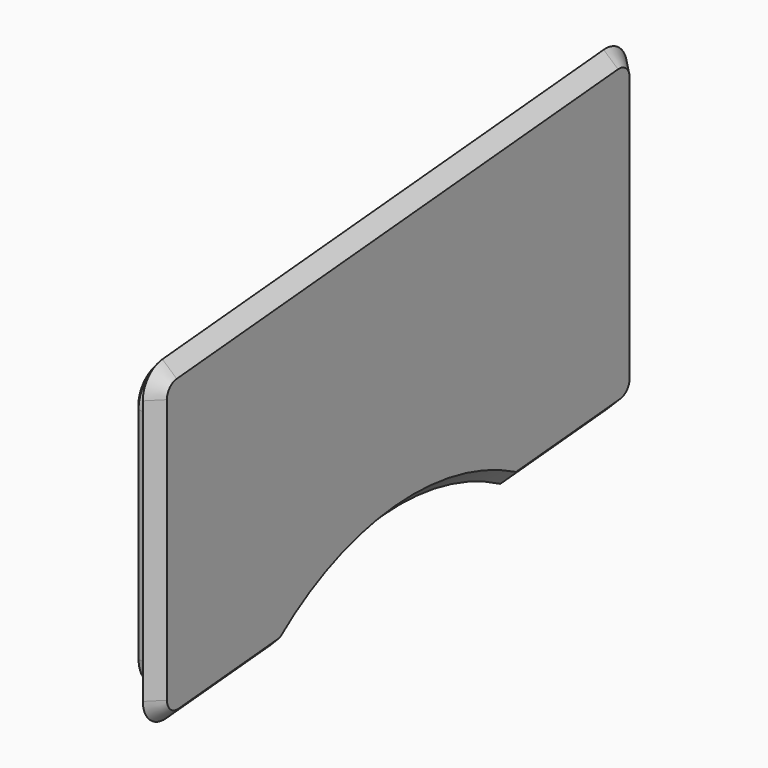
from build123d import *

# Parameters (mm, degrees)
F1_DEPTH     = 3
F2_DEPTH     = 8
F3_R         = 8
F4_T4_DEPTH  = 113.9006842239
F4_T9_ANGLE  = 95
F4_T14_ANGLE = 85
F4_T19_DEPTH = 49.1871720396
F4_T24_ANGLE = 95
F4_T29_DEPTH = 20.662188907
F4_T34_ANGLE = 31.4669762933
F4_T39_ANGLE = 62.9339525865
F4_T44_ANGLE = 31.4669762933
F4_T49_DEPTH = 22.2455379196
F4_T54_ANGLE = 85
F4_T59_DEPTH = 49.1871720396
F5_SIZE      = 1
F6_T1_DEPTH  = 123.9388825993
F6_T3_DEPTH  = 59.2253704151
F6_T5_DEPTH  = 42.8508484491
F6_T7_DEPTH  = 59.2253704151
F6_T9_DEPTH  = 43.5593108265
F6_T12_ANGLE = 96.9904356043
F6_T14_ANGLE = 95
F6_T16_ANGLE = 85
F6_T18_ANGLE = 95
F6_T20_ANGLE = 85


# Not quite as in the source:
# - a fillet or chamfer that OpenCascade refuses, or shapes differently, is made with other operations: its cross-section is extruded or revolved along the edge and cut away or added


with BuildPart() as f1:
    # F0 (on Right) → F1 (new body)
    with BuildSketch(Plane.YZ):
        with BuildLine():
            Line((-76.6886542646, 55.3186824411), (-76.6886542646, -19.9678053747))
            Line((-76.6886542646, -19.9678053747), (-38.1131050777, -16.5928821315))
            ThreePointArc((-38.1131050777, -16.5928821315), (-7.4822201157, -3.8748285682), (24.8917797013, -11.0806689666))
            Line((24.8917797013, -11.0806689666), (62.7786034683, -7.76600139))
            Line((62.7786034683, -7.76600139), (62.7786034683, 67.5204864257))
            Line((62.7786034683, 67.5204864257), (-76.6886542646, 55.3186824411))
        make_face()
        with BuildLine():
            Line((-40.0864817191, -11.7464310288), (-71.6886542646, -14.5112628693))
            Line((-71.6886542646, -14.5112628693), (-71.6886542646, 50.737026571))
            Line((-71.6886542646, 50.737026571), (57.7786034683, 62.0639439204))
            Line((57.7786034683, 62.0639439204), (57.7786034683, -3.1843455199))
            Line((57.7786034683, -3.1843455199), (25.9935989152, -5.9651730884))
            ThreePointArc((25.9935989152, -5.9651730884), (-7.9179988294, 1.1061449223), (-40.0864817191, -11.7464310288))
        make_face(mode=Mode.SUBTRACT)
        with BuildLine():
            Line((-71.6886542646, 50.737026571), (-71.6886542646, -14.5112628693))
            Line((-71.6886542646, -14.5112628693), (-40.0864817191, -11.7464310288))
            ThreePointArc((-40.0864817191, -11.7464310288), (-7.9179988294, 1.1061449223), (25.9935989152, -5.9651730884))
            Line((25.9935989152, -5.9651730884), (57.7786034683, -3.1843455199))
            Line((57.7786034683, -3.1843455199), (57.7786034683, 62.0639439204))
            Line((57.7786034683, 62.0639439204), (-71.6886542646, 50.737026571))
        make_face()
    extrude(amount=-F1_DEPTH)

    # F0 (on Right) → F2 (join)
    with BuildSketch(Plane.YZ):
        with BuildLine():
            Line((-71.6886542646, 50.737026571), (-71.6886542646, -14.5112628693))
            Line((-71.6886542646, -14.5112628693), (-40.0864817191, -11.7464310288))
            ThreePointArc((-40.0864817191, -11.7464310288), (-7.9179988294, 1.1061449223), (25.9935989152, -5.9651730884))
            Line((25.9935989152, -5.9651730884), (57.7786034683, -3.1843455199))
            Line((57.7786034683, -3.1843455199), (57.7786034683, 62.0639439204))
            Line((57.7786034683, 62.0639439204), (-71.6886542646, 50.737026571))
        make_face()
    extrude(amount=-F2_DEPTH)

    # F3
    f3_edges = [f1.edges().sort_by_distance(p)[0] for p in [
        (-5.5, 57.778603, 62.063944),
        (-5.5, -71.688654, 50.737027),
        (-5.5, -71.688654, -14.511263),
        (-5.5, -40.086482, -11.746431),
        (-5.5, 25.993599, -5.965173),
        (-5.5, 57.778603, -3.184346),
        (-1.5, -76.688654, 55.318682),
        (-1.5, -76.688654, -19.967805),
        (-1.5, 62.778603, -7.766001),
        (-1.5, 62.778603, 67.520486),
    ]]
    fillet(f3_edges, radius=F3_R)

    # F4: chamfer of 1 x 6 on 1 edges, made by hand


with BuildPart() as f4_tool2:
    # F4_s3 → F4_t4 (new body)
    with BuildSketch(Plane(origin=(0, 54.0311094993, 4.7271095589), x_dir=(1, 0, 0), z_dir=(0, -0.9961946981, -0.0871557427))):
        Polygon((-2, 56.792034776), (-8, 55.792034776), (-8, 56.792034776), align=None)
    extrude(amount=F4_T4_DEPTH)

    split(bisect_by=Plane.YZ.offset(-3), keep=Keep.BOTTOM)


with BuildPart() as f1_1:
    add(f1.part)

    # F4_t1: cut F4_tool2
    add(f4_tool2.part, mode=Mode.SUBTRACT)


with BuildPart() as f4_tool7:
    # F4_s8 → F4_t9 (revolve)
    with BuildSketch(Plane.XY.offset(53.3334759118)):
        Polygon((-2, 57.7786034683), (-8, 56.7786034683), (-8, 57.7786034683), align=None)
    revolve(axis=Axis((-8, 49.7786034683, 53.3334759118), (1, 0, 0)), revolution_arc=F4_T9_ANGLE)

    split(bisect_by=Plane.YZ.offset(-3), keep=Keep.BOTTOM)


with BuildPart() as f1_2:
    add(f1_1.part)

    # F4_t6: cut F4_tool7
    add(f4_tool7.part, mode=Mode.SUBTRACT)


with BuildPart() as f4_tool12:
    # F4_s13 → F4_t14 (revolve)
    with BuildSketch(Plane.XY.offset(43.4063771788)):
        Polygon((-2, -71.6886542646), (-8, -70.6886542646), (-8, -71.6886542646), align=None)
    revolve(axis=Axis((-8, -63.6886542646, 43.4063771788), (-1, 0, 0)), revolution_arc=F4_T14_ANGLE)

    split(bisect_by=Plane.YZ.offset(-3), keep=Keep.BOTTOM)


with BuildPart() as f1_3:
    add(f1_2.part)

    # F4_t11: cut F4_tool12
    add(f4_tool12.part, mode=Mode.SUBTRACT)


with BuildPart() as f4_tool17:
    # F4_s18 → F4_t19 (new body)
    with BuildSketch(Plane.XY.offset(43.4063771788)):
        Polygon((-2, -71.6886542646), (-8, -70.6886542646), (-8, -71.6886542646), align=None)
    extrude(amount=-F4_T19_DEPTH)

    split(bisect_by=Plane.YZ.offset(-3), keep=Keep.BOTTOM)


with BuildPart() as f1_4:
    add(f1_3.part)

    # F4_t16: cut F4_tool17
    add(f4_tool17.part, mode=Mode.SUBTRACT)


with BuildPart() as f4_tool22:
    # F4_s23 → F4_t24 (revolve)
    with BuildSketch(Plane.XY.offset(-5.7807948608)):
        Polygon((-2, -71.6886542646), (-8, -70.6886542646), (-8, -71.6886542646), align=None)
    revolve(axis=Axis((-8, -63.6886542646, -5.7807948608), (1, 0, 0)), revolution_arc=F4_T24_ANGLE)

    split(bisect_by=Plane.YZ.offset(-3), keep=Keep.BOTTOM)


with BuildPart() as f1_5:
    add(f1_4.part)

    # F4_t21: cut F4_tool22
    add(f4_tool22.part, mode=Mode.SUBTRACT)


with BuildPart() as f4_tool27:
    # F4_s28 → F4_t29 (new body)
    with BuildSketch(Plane(origin=(0, -63.7067796281, -5.5736210072), x_dir=(1, 0, 0), z_dir=(0, 0.9961946981, 0.0871557427))):
        Polygon((-2, 8.207965224), (-8, 7.207965224), (-8, 8.207965224), align=None)
    extrude(amount=F4_T29_DEPTH)

    split(bisect_by=Plane.YZ.offset(-3), keep=Keep.BOTTOM)


with BuildPart() as f1_6:
    add(f1_5.part)

    # F4_t26: cut F4_tool27
    add(f4_tool27.part, mode=Mode.SUBTRACT)


with BuildPart() as f4_tool32:
    # F4_s33 → F4_t34 (revolve)
    with BuildSketch(Plane(origin=(0, -43.123216588, -3.7727925862), x_dir=(1, 0, 0), z_dir=(0, -0.9961946981, -0.0871557427))):
        Polygon((-2, -8.207965224), (-8, -7.207965224), (-8, -8.207965224), align=None)
    revolve(axis=Axis((-8, -43.1050912244, -3.9799664398), (1, 0, 0)), revolution_arc=F4_T34_ANGLE)

    split(bisect_by=Plane.YZ.offset(-3), keep=Keep.BOTTOM)


with BuildPart() as f1_7:
    add(f1_6.part)

    # F4_t31: cut F4_tool32
    add(f4_tool32.part, mode=Mode.SUBTRACT)


with BuildPart() as f4_tool37:
    # F4_s38 → F4_t39 (revolve)
    with BuildSketch(Plane(origin=(0, -29.7800133865, -22.0094994379), x_dir=(1, 0, 0), z_dir=(0, -0.8041995665, -0.5943593671))):
        Polygon((-2, 14.4192274514), (-8, 15.4192274514), (-8, 14.4192274514), align=None)
    revolve(axis=Axis((-8, -2.6886542646, -58.6655369632), (-1, 0, 0)), revolution_arc=F4_T39_ANGLE)

    split(bisect_by=Plane.YZ.offset(-3), keep=Keep.BOTTOM)


with BuildPart() as f1_8:
    add(f1_7.part)

    # F4_t36: cut F4_tool37
    add(f4_tool37.part, mode=Mode.SUBTRACT)


with BuildPart() as f4_tool42:
    # F4_s43 → F4_t44 (revolve)
    with BuildSketch(Plane(origin=(0, 21.2512251902, -10.5801809941), x_dir=(1, 0, 0), z_dir=(0, -0.895191389, 0.4456819235))):
        Polygon((-2, 6.2848318723), (-8, 7.2848318723), (-8, 6.2848318723), align=None)
    revolve(axis=Axis((-8, 27.6177165365, 2.207477492), (1, 0, 0)), revolution_arc=F4_T44_ANGLE)

    split(bisect_by=Plane.YZ.offset(-3), keep=Keep.BOTTOM)


with BuildPart() as f1_9:
    add(f1_8.part)

    # F4_t41: cut F4_tool42
    add(f4_tool42.part, mode=Mode.SUBTRACT)


with BuildPart() as f4_tool47:
    # F4_s48 → F4_t49 (new body)
    with BuildSketch(Plane(origin=(0, 27.599591173, 2.4146513456), x_dir=(1, 0, 0), z_dir=(0, 0.9961946981, 0.0871557427))):
        Polygon((-2, 8.207965224), (-8, 7.207965224), (-8, 8.207965224), align=None)
    extrude(amount=F4_T49_DEPTH)

    split(bisect_by=Plane.YZ.offset(-3), keep=Keep.BOTTOM)


with BuildPart() as f1_10:
    add(f1_9.part)

    # F4_t46: cut F4_tool47
    add(f4_tool47.part, mode=Mode.SUBTRACT)


with BuildPart() as f4_tool52:
    # F4_s53 → F4_t54 (revolve)
    with BuildSketch(Plane(origin=(0, 49.7604781047, 4.3534777258), x_dir=(1, 0, 0), z_dir=(0, -0.9961946981, -0.0871557427))):
        Polygon((-2, -8.207965224), (-8, -7.207965224), (-8, -8.207965224), align=None)
    revolve(axis=Axis((-8, 49.7786034683, 4.1463038722), (1, 0, 0)), revolution_arc=F4_T54_ANGLE)

    split(bisect_by=Plane.YZ.offset(-3), keep=Keep.BOTTOM)


with BuildPart() as f1_11:
    add(f1_10.part)

    # F4_t51: cut F4_tool52
    add(f4_tool52.part, mode=Mode.SUBTRACT)


with BuildPart() as f4_tool57:
    # F4_s58 → F4_t59 (new body)
    with BuildSketch(Plane.XY.offset(4.1463038722)):
        Polygon((-2, 57.7786034683), (-8, 56.7786034683), (-8, 57.7786034683), align=None)
    extrude(amount=F4_T59_DEPTH)

    split(bisect_by=Plane.YZ.offset(-3), keep=Keep.BOTTOM)


with BuildPart() as f1_12:
    add(f1_11.part)

    # F4_t56: cut F4_tool57
    add(f4_tool57.part, mode=Mode.SUBTRACT)

    # F5
    f5_edges = [f1_12.edges().sort_by_distance(p)[0] for p in [
        (-8, -7.565116, 55.343289),
        (-8, -68.849596, 48.135509),
        (-8, 54.507735, 58.494417),
        (-8, 54.939545, -0.582828),
        (-8, 39.30825, -3.796472),
        (-8, 26.31403, -4.670051),
        (-8, -8.005155, 2.10234),
        (-8, -40.626941, -10.526627),
        (-8, -52.786783, -11.853744),
        (-8, -68.417786, -10.941736),
        (-8, -70.688654, 18.812791),
        (-8, 56.778603, 28.73989),
    ]]
    chamfer(f5_edges, length=F5_SIZE)

    # F6: chamfer of 5 on 2 edges, made by hand

    # F6_s2 → F6_t1 (cut)
    with BuildSketch(Plane(origin=(0, 59.4668882131, 5.2026785738), x_dir=(1, 0, 0), z_dir=(0, -0.9961946981, -0.0871557427))):
        Polygon((-5, 61.792034776), (0, 56.792034776), (0, 61.792034776), align=None)
    extrude(amount=F6_T1_DEPTH, mode=Mode.SUBTRACT)

    # F6_s4 → F6_t3 (cut)
    with BuildSketch(Plane.XY.offset(-11.2373373661)):
        Polygon((-5, -76.6886542646), (0, -71.6886542646), (0, -76.6886542646), align=None)
    extrude(amount=F6_T3_DEPTH, mode=Mode.SUBTRACT)

    # F6_s6 → F6_t5 (cut)
    with BuildSketch(Plane(origin=(0, -69.1425583419, -6.0491900221), x_dir=(1, 0, 0), z_dir=(0, 0.9961946981, 0.0871557427))):
        Polygon((-5, 13.207965224), (0, 8.207965224), (0, 13.207965224), align=None)
    extrude(amount=F6_T5_DEPTH, mode=Mode.SUBTRACT)

    # F6_s8 → F6_t7 (cut)
    with BuildSketch(Plane.XY.offset(-0.4353519979)):
        Polygon((-5, 62.7786034683), (0, 57.7786034683), (0, 62.7786034683), align=None)
    extrude(amount=F6_T7_DEPTH, mode=Mode.SUBTRACT)

    # F6_s10 → F6_t9 (cut)
    with BuildSketch(Plane(origin=(0, 10.9311448931, 0.9563512575), x_dir=(1, 0, 0), z_dir=(0, 0.9961946981, 0.0871557427))):
        Polygon((-5, 13.207965224), (0, 8.207965224), (0, 13.207965224), align=None)
    extrude(amount=F6_T9_DEPTH, mode=Mode.SUBTRACT)

    # F6_s11 → F6_t12 (revolve, cut)
    with BuildSketch(Plane(origin=(0, -29.0039957446, -39.1898093404), x_dir=(1, 0, 0), z_dir=(0, -0.5948898787, -0.8038072109))):
        Polygon((-5, 22.2616255192), (0, 27.2616255192), (0, 22.2616255192), align=None)
    revolve(axis=Axis((0, -2.6886542646, -58.6655369632), (-1, 0, 0)), revolution_arc=F6_T12_ANGLE, mode=Mode.SUBTRACT)

    # F6_s13 → F6_t14 (revolve, cut)
    with BuildSketch(Plane(origin=(0, 59.4668882131, 5.2026785738), x_dir=(1, 0, 0), z_dir=(0, -0.9961946981, -0.0871557427))):
        Polygon((-5, 61.792034776), (0, 56.792034776), (0, 61.792034776), align=None)
    revolve(axis=Axis((0, 54.7786034683, 58.7900184172), (-1, 0, 0)), revolution_arc=F6_T14_ANGLE, mode=Mode.SUBTRACT)

    # F6_s15 → F6_t16 (revolve, cut)
    with BuildSketch(Plane.XY.offset(47.9880330489)):
        Polygon((-5, -76.6886542646), (0, -71.6886542646), (0, -76.6886542646), align=None)
    revolve(axis=Axis((0, -68.6886542646, 47.9880330489), (-1, 0, 0)), revolution_arc=F6_T16_ANGLE, mode=Mode.SUBTRACT)

    # F6_s17 → F6_t18 (revolve, cut)
    with BuildSketch(Plane.XY.offset(-11.2373373661)):
        Polygon((-5, -76.6886542646), (0, -71.6886542646), (0, -76.6886542646), align=None)
    revolve(axis=Axis((0, -68.6886542646, -11.2373373661), (1, 0, 0)), revolution_arc=F6_T18_ANGLE, mode=Mode.SUBTRACT)

    # F6_s19 → F6_t20 (revolve, cut)
    with BuildSketch(Plane.XY.offset(-0.4353519979)):
        Polygon((-5, 62.7786034683), (0, 57.7786034683), (0, 62.7786034683), align=None)
    revolve(axis=Axis((0, 54.7786034683, -0.4353519979), (-1, 0, 0)), revolution_arc=F6_T20_ANGLE, mode=Mode.SUBTRACT)


solid = f1_12.part
